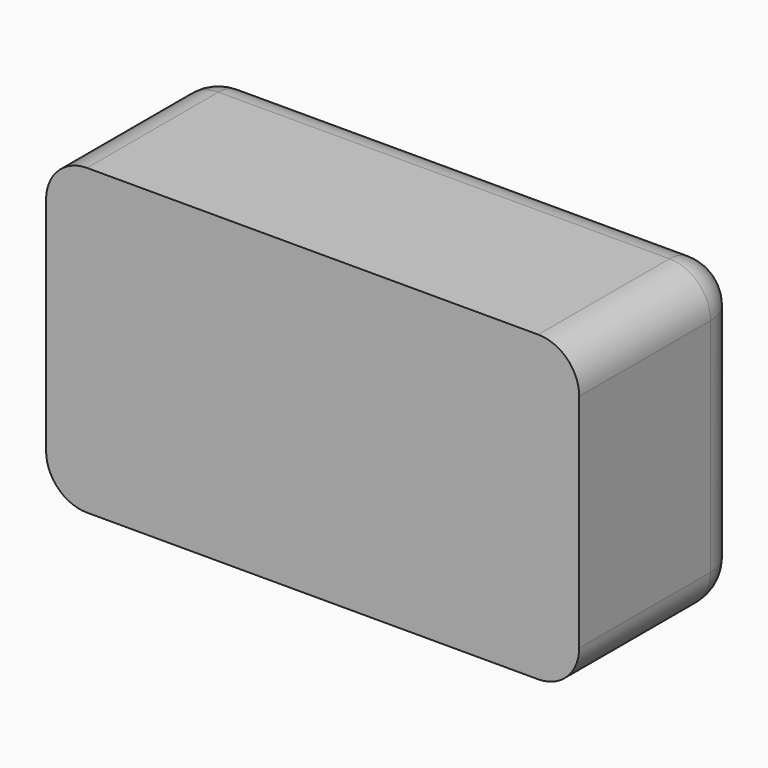
from build123d import *

# Parameters (mm, degrees)
F0_W        = 65
F0_H        = 37
F1_DEPTH    = 25
F2_R        = 5
F3_T1_DEPTH = 32.5
F3_S5_W     = 5
F3_S5_H     = 5
F3_T6_DEPTH = 5


# Not quite as in the source:
# - a fillet or chamfer that OpenCascade refuses, or shapes differently, is made with other operations: its cross-section is extruded or revolved along the edge and cut away or added


with BuildPart() as f1:
    # F0 (on Front) → F1 (new body)
    with BuildSketch(Plane.XZ):
        Rectangle(F0_W, F0_H)
    extrude(amount=F1_DEPTH)

    # F2
    f2_edges = [f1.edges().sort_by_distance(p)[0] for p in [
        (-32.5, -12.5, 18.5),
        (-32.5, -12.5, -18.5),
        (0, 0, 18.5),
        (-32.5, 0, 0),
        (32.5, 0, 0),
        (32.5, -12.5, -18.5),
        (0, 0, -18.5),
    ]]
    fillet(f2_edges, radius=F2_R)

    # F3: fillet of radius 5 on 1 edges, made by hand

    # F3_s2 → F3_t1 (cut)
    with BuildSketch(Plane.XZ.offset(5)):
        with BuildLine():
            ThreePointArc((27.5, 18.5), (31.0355339059, 17.0355339059), (32.5, 13.5))
            Line((32.5, 13.5), (32.5, 18.5))
            Line((32.5, 18.5), (27.5, 18.5))
        make_face()
    extrude(amount=F3_T1_DEPTH, mode=Mode.SUBTRACT)


with BuildPart() as f3_tool4:
    # F3_s5 → F3_t6 (new body)
    with BuildSketch(Plane.XY.offset(13.5)):
        with Locations((30, -2.5)):
            Rectangle(F3_S5_W, F3_S5_H)
    extrude(amount=F3_T6_DEPTH)

    # F3_s7 → F3_t8 (revolve, cut)
    with BuildSketch(Plane(origin=(27.5, -5, 13.5), x_dir=(-0.7071067812, -0.7071067812, 0), z_dir=(-0.7071067812, 0.7071067812, 0))):
        with BuildLine():
            ThreePointArc((0, -5), (5, 0), (0, 5))
            Line((0, 5), (0, -5))
        make_face()
    revolve(axis=Axis((27.5, -5, 13.5), (0, 0, 1)), mode=Mode.SUBTRACT)


with BuildPart() as f1_1:
    add(f1.part)

    # F3_t3: cut F3_tool4
    add(f3_tool4.part, mode=Mode.SUBTRACT)


solid = f1_1.part
